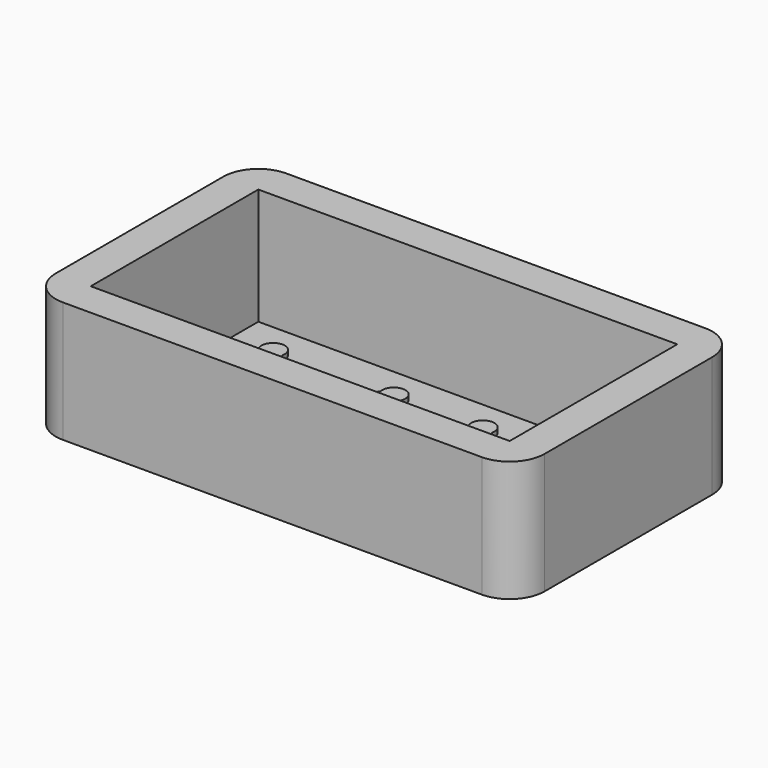
from build123d import *

# Parameters (mm, degrees)
F0_W     = 17.75
F0_H     = 18
F0_W_2   = 0.25
F1_DEPTH = 0.4
F2_DEPTH = 10
F3_DEPTH = 0.2
F4_DEPTH = 0.4


# Not quite as in the source:
# - a feature names something its author has since deleted; it is built from what else it names


with BuildPart() as f1:
    # F0 (on Top) → F1 (new body)
    with BuildSketch(Plane.XY):
        with BuildLine():
            Line((36, 21), (0, 21))
            ThreePointArc((0, 21), (-2.1213203436, 20.1213203436), (-3, 18))
            Line((-3, 18), (-3, 0))
            ThreePointArc((-3, 0), (-2.1213203436, -2.1213203436), (0, -3))
            Line((0, -3), (36, -3))
            ThreePointArc((36, -3), (38.1213203436, -2.1213203436), (39, 0))
            Line((39, 0), (39, 18))
            ThreePointArc((39, 18), (38.1213203436, 20.1213203436), (36, 21))
        make_face()
        Polygon((0, 0), (0, 18), (17.75, 18), (18, 18), (18.25, 18), (36, 18), (36, 0), (18.25, 0), (18, 0), (17.75, 0), align=None, mode=Mode.SUBTRACT)
        with Locations((8.875, 9)):
            Rectangle(F0_W, F0_H)
        with BuildLine():
            Line((9.6533412223, 11.6952957055), (9.9919033945, 10.9452957055))
            Line((9.9919033945, 10.9452957055), (10.3304655668, 11.6952957055))
            Line((10.3304655668, 11.6952957055), (10.9904227081, 12.3580254744))
            Line((10.9904227081, 12.3580254744), (13.2079580316, 14.5755632326))
            ThreePointArc((13.2079580316, 14.5755632326), (14.8809903029, 15.5414897832), (13.9150646707, 13.8684569817))
            Line((13.9150646707, 13.8684569817), (10.9919033945, 10.9452957055))
            Line((10.9919033945, 10.9452957055), (10.9919033945, 9.4452957055))
            Line((10.9919033945, 9.4452957055), (13.6148667214, 9.4452957055))
            ThreePointArc((13.6148667214, 9.4452957055), (13.70376764, 9.5296679116), (13.8052234095, 9.5984339593))
            ThreePointArc((13.8052234095, 9.5984339593), (14.9138690208, 8.823141097), (13.6148667214, 8.4452957055))
            Line((13.6148667214, 8.4452957055), (10.9919033945, 8.4452957055))
            Line((10.9919033945, 8.4452957055), (10.9919033945, 6.9452957055))
            Line((10.9919033945, 6.9452957055), (13.9150646707, 4.0221344294))
            ThreePointArc((13.9150646707, 4.0221344294), (14.8809903029, 2.3491016278), (13.2079580316, 3.3150281785))
            Line((13.2079580316, 3.3150281785), (10.9904227081, 5.5325659367))
            Line((10.9904227081, 5.5325659367), (10.3304655668, 6.1952957055))
            Line((10.3304655668, 6.1952957055), (9.9919033945, 6.9452957055))
            Line((9.9919033945, 6.9452957055), (9.6533412223, 6.1952957055))
            ThreePointArc((9.6533412223, 6.1952957055), (8.9919033945, 4.4452957055), (8.3304655668, 6.1952957055))
            Line((8.3304655668, 6.1952957055), (7.9919033945, 6.9452957055))
            Line((7.9919033945, 6.9452957055), (7.6533412223, 6.1952957055))
            Line((7.6533412223, 6.1952957055), (6.993384081, 5.5325659367))
            Line((6.993384081, 5.5325659367), (4.7758487575, 3.3150281785))
            ThreePointArc((4.7758487575, 3.3150281785), (3.1028164862, 2.3491016278), (4.0687421184, 4.0221344294))
            Line((4.0687421184, 4.0221344294), (6.9919033945, 6.9452957055))
            Line((6.9919033945, 6.9452957055), (6.9919033945, 8.4452957055))
            Line((6.9919033945, 8.4452957055), (4.3689400677, 8.4452957055))
            ThreePointArc((4.3689400677, 8.4452957055), (3.0699377683, 8.823141097), (4.1785833795, 9.5984339593))
            ThreePointArc((4.1785833795, 9.5984339593), (4.2800391491, 9.5296679116), (4.3689400677, 9.4452957055))
            Line((4.3689400677, 9.4452957055), (6.9919033945, 9.4452957055))
            Line((6.9919033945, 9.4452957055), (6.9919033945, 10.9452957055))
            Line((6.9919033945, 10.9452957055), (4.0687421184, 13.8684569817))
            ThreePointArc((4.0687421184, 13.8684569817), (3.1028164862, 15.5414897832), (4.7758487575, 14.5755632326))
            Line((4.7758487575, 14.5755632326), (6.993384081, 12.3580254744))
            Line((6.993384081, 12.3580254744), (7.6533412223, 11.6952957055))
            Line((7.6533412223, 11.6952957055), (7.9919033945, 10.9452957055))
            Line((7.9919033945, 10.9452957055), (8.3304655668, 11.6952957055))
            ThreePointArc((8.3304655668, 11.6952957055), (8.9919033945, 13.4452957055), (9.6533412223, 11.6952957055))
        make_face(mode=Mode.SUBTRACT)
        with Locations((27.125, 9)):
            Rectangle(F0_W, F0_H)
        with BuildLine():
            Line((27.6695344332, 11.6952957055), (28.0080966055, 10.9452957055))
            Line((28.0080966055, 10.9452957055), (28.3466587777, 11.6952957055))
            Line((28.3466587777, 11.6952957055), (29.006615919, 12.3580254744))
            Line((29.006615919, 12.3580254744), (31.2241512425, 14.5755632326))
            ThreePointArc((31.2241512425, 14.5755632326), (32.8971835138, 15.5414897832), (31.9312578816, 13.8684569817))
            Line((31.9312578816, 13.8684569817), (29.0080966055, 10.9452957055))
            Line((29.0080966055, 10.9452957055), (29.0080966055, 9.4452957055))
            Line((29.0080966055, 9.4452957055), (31.6310599323, 9.4452957055))
            ThreePointArc((31.6310599323, 9.4452957055), (31.7199608509, 9.5296679116), (31.8214166205, 9.5984339593))
            ThreePointArc((31.8214166205, 9.5984339593), (32.9300622317, 8.823141097), (31.6310599323, 8.4452957055))
            Line((31.6310599323, 8.4452957055), (29.0080966055, 8.4452957055))
            Line((29.0080966055, 8.4452957055), (29.0080966055, 6.9452957055))
            Line((29.0080966055, 6.9452957055), (31.9312578816, 4.0221344294))
            ThreePointArc((31.9312578816, 4.0221344294), (32.8971835138, 2.3491016278), (31.2241512425, 3.3150281785))
            Line((31.2241512425, 3.3150281785), (29.006615919, 5.5325659367))
            Line((29.006615919, 5.5325659367), (28.3466587777, 6.1952957055))
            Line((28.3466587777, 6.1952957055), (28.0080966055, 6.9452957055))
            Line((28.0080966055, 6.9452957055), (27.6695344332, 6.1952957055))
            ThreePointArc((27.6695344332, 6.1952957055), (27.0080966055, 4.4452957055), (26.3466587777, 6.1952957055))
            Line((26.3466587777, 6.1952957055), (26.0080966055, 6.9452957055))
            Line((26.0080966055, 6.9452957055), (25.6695344332, 6.1952957055))
            Line((25.6695344332, 6.1952957055), (25.0095772919, 5.5325659367))
            Line((25.0095772919, 5.5325659367), (22.7920419684, 3.3150281785))
            ThreePointArc((22.7920419684, 3.3150281785), (21.1190096971, 2.3491016278), (22.0849353293, 4.0221344294))
            Line((22.0849353293, 4.0221344294), (25.0080966055, 6.9452957055))
            Line((25.0080966055, 6.9452957055), (25.0080966055, 8.4452957055))
            Line((25.0080966055, 8.4452957055), (22.3851332786, 8.4452957055))
            ThreePointArc((22.3851332786, 8.4452957055), (21.0861309792, 8.823141097), (22.1947765905, 9.5984339593))
            ThreePointArc((22.1947765905, 9.5984339593), (22.29623236, 9.5296679116), (22.3851332786, 9.4452957055))
            Line((22.3851332786, 9.4452957055), (25.0080966055, 9.4452957055))
            Line((25.0080966055, 9.4452957055), (25.0080966055, 10.9452957055))
            Line((25.0080966055, 10.9452957055), (22.0849353293, 13.8684569817))
            ThreePointArc((22.0849353293, 13.8684569817), (21.1190096971, 15.5414897832), (22.7920419684, 14.5755632326))
            Line((22.7920419684, 14.5755632326), (25.0095772919, 12.3580254744))
            Line((25.0095772919, 12.3580254744), (25.6695344332, 11.6952957055))
            Line((25.6695344332, 11.6952957055), (26.0080966055, 10.9452957055))
            Line((26.0080966055, 10.9452957055), (26.3466587777, 11.6952957055))
            ThreePointArc((26.3466587777, 11.6952957055), (27.0080966055, 13.4452957055), (27.6695344332, 11.6952957055))
        make_face(mode=Mode.SUBTRACT)
        with BuildLine():
            Line((26.0080966055, 8.9452957055), (26.0080966055, 10.9452957055))
            Line((26.0080966055, 10.9452957055), (25.6695344332, 11.6952957055))
            Line((25.6695344332, 11.6952957055), (25.0095772919, 12.3580254744))
            Line((25.0095772919, 12.3580254744), (22.7920419684, 14.5755632326))
            ThreePointArc((22.7920419684, 14.5755632326), (21.1190096971, 15.5414897832), (22.0849353293, 13.8684569817))
            Line((22.0849353293, 13.8684569817), (25.0080966055, 10.9452957055))
            Line((25.0080966055, 10.9452957055), (25.0080966055, 9.4452957055))
            Line((25.0080966055, 9.4452957055), (25.0080966055, 8.9452957055))
            Line((25.0080966055, 8.9452957055), (25.0080966055, 8.4452957055))
            Line((25.0080966055, 8.4452957055), (25.0080966055, 6.9452957055))
            Line((25.0080966055, 6.9452957055), (22.0849353293, 4.0221344294))
            ThreePointArc((22.0849353293, 4.0221344294), (21.1190096971, 2.3491016278), (22.7920419684, 3.3150281785))
            Line((22.7920419684, 3.3150281785), (25.0095772919, 5.5325659367))
            Line((25.0095772919, 5.5325659367), (25.6695344332, 6.1952957055))
            Line((25.6695344332, 6.1952957055), (26.0080966055, 6.9452957055))
            Line((26.0080966055, 6.9452957055), (26.0080966055, 8.9452957055))
        make_face()
        with BuildLine():
            Line((28.3466587777, 11.6952957055), (28.0080966055, 10.9452957055))
            Line((28.0080966055, 10.9452957055), (28.0080966055, 8.9452957055))
            Line((28.0080966055, 8.9452957055), (28.0080966055, 6.9452957055))
            Line((28.0080966055, 6.9452957055), (28.3466587777, 6.1952957055))
            Line((28.3466587777, 6.1952957055), (29.006615919, 5.5325659367))
            Line((29.006615919, 5.5325659367), (31.2241512425, 3.3150281785))
            ThreePointArc((31.2241512425, 3.3150281785), (32.8971835138, 2.3491016278), (31.9312578816, 4.0221344294))
            Line((31.9312578816, 4.0221344294), (29.0080966055, 6.9452957055))
            Line((29.0080966055, 6.9452957055), (29.0080966055, 8.4452957055))
            Line((29.0080966055, 8.4452957055), (29.0080966055, 8.9452957055))
            Line((29.0080966055, 8.9452957055), (29.0080966055, 9.4452957055))
            Line((29.0080966055, 9.4452957055), (29.0080966055, 10.9452957055))
            Line((29.0080966055, 10.9452957055), (31.9312578816, 13.8684569817))
            ThreePointArc((31.9312578816, 13.8684569817), (32.8971835138, 15.5414897832), (31.2241512425, 14.5755632326))
            Line((31.2241512425, 14.5755632326), (29.006615919, 12.3580254744))
            Line((29.006615919, 12.3580254744), (28.3466587777, 11.6952957055))
        make_face()
        with BuildLine():
            Line((7.9919033945, 8.9452957055), (7.9919033945, 10.9452957055))
            Line((7.9919033945, 10.9452957055), (7.6533412223, 11.6952957055))
            Line((7.6533412223, 11.6952957055), (6.993384081, 12.3580254744))
            Line((6.993384081, 12.3580254744), (4.7758487575, 14.5755632326))
            ThreePointArc((4.7758487575, 14.5755632326), (3.1028164862, 15.5414897832), (4.0687421184, 13.8684569817))
            Line((4.0687421184, 13.8684569817), (6.9919033945, 10.9452957055))
            Line((6.9919033945, 10.9452957055), (6.9919033945, 9.4452957055))
            Line((6.9919033945, 9.4452957055), (6.9919033945, 8.9452957055))
            Line((6.9919033945, 8.9452957055), (6.9919033945, 8.4452957055))
            Line((6.9919033945, 8.4452957055), (6.9919033945, 6.9452957055))
            Line((6.9919033945, 6.9452957055), (4.0687421184, 4.0221344294))
            ThreePointArc((4.0687421184, 4.0221344294), (3.1028164862, 2.3491016278), (4.7758487575, 3.3150281785))
            Line((4.7758487575, 3.3150281785), (6.993384081, 5.5325659367))
            Line((6.993384081, 5.5325659367), (7.6533412223, 6.1952957055))
            Line((7.6533412223, 6.1952957055), (7.9919033945, 6.9452957055))
            Line((7.9919033945, 6.9452957055), (7.9919033945, 8.9452957055))
        make_face()
        with BuildLine():
            Line((9.9919033945, 10.9452957055), (9.9919033945, 8.9452957055))
            Line((9.9919033945, 8.9452957055), (9.9919033945, 6.9452957055))
            Line((9.9919033945, 6.9452957055), (10.3304655668, 6.1952957055))
            Line((10.3304655668, 6.1952957055), (10.9904227081, 5.5325659367))
            Line((10.9904227081, 5.5325659367), (13.2079580316, 3.3150281785))
            ThreePointArc((13.2079580316, 3.3150281785), (14.8809903029, 2.3491016278), (13.9150646707, 4.0221344294))
            Line((13.9150646707, 4.0221344294), (10.9919033945, 6.9452957055))
            Line((10.9919033945, 6.9452957055), (10.9919033945, 8.4452957055))
            Line((10.9919033945, 8.4452957055), (10.9919033945, 8.9452957055))
            Line((10.9919033945, 8.9452957055), (10.9919033945, 9.4452957055))
            Line((10.9919033945, 9.4452957055), (10.9919033945, 10.9452957055))
            Line((10.9919033945, 10.9452957055), (13.9150646707, 13.8684569817))
            ThreePointArc((13.9150646707, 13.8684569817), (14.8809903029, 15.5414897832), (13.2079580316, 14.5755632326))
            Line((13.2079580316, 14.5755632326), (10.9904227081, 12.3580254744))
            Line((10.9904227081, 12.3580254744), (10.3304655668, 11.6952957055))
            Line((10.3304655668, 11.6952957055), (9.9919033945, 10.9452957055))
        make_face()
        with BuildLine():
            Line((28.0080966055, 8.9452957055), (28.0080966055, 10.9452957055))
            Line((28.0080966055, 10.9452957055), (27.6695344332, 11.6952957055))
            ThreePointArc((27.6695344332, 11.6952957055), (27.0080966055, 13.4452957055), (26.3466587777, 11.6952957055))
            Line((26.3466587777, 11.6952957055), (26.0080966055, 10.9452957055))
            Line((26.0080966055, 10.9452957055), (26.0080966055, 8.9452957055))
            Line((26.0080966055, 8.9452957055), (26.0080966055, 6.9452957055))
            Line((26.0080966055, 6.9452957055), (26.3466587777, 6.1952957055))
            ThreePointArc((26.3466587777, 6.1952957055), (27.0080966055, 4.4452957055), (27.6695344332, 6.1952957055))
            Line((27.6695344332, 6.1952957055), (28.0080966055, 6.9452957055))
            Line((28.0080966055, 6.9452957055), (28.0080966055, 8.9452957055))
        make_face()
        with BuildLine():
            ThreePointArc((27.0080966055, 9.1952957055), (27.1848733008, 9.1220724008), (27.2580966055, 8.9452957055))
            ThreePointArc((27.2580966055, 8.9452957055), (27.1848733008, 8.7685190102), (27.0080966055, 8.6952957055))
            ThreePointArc((27.0080966055, 8.6952957055), (26.7580966055, 8.9452957055), (27.0080966055, 9.1952957055))
        make_face(mode=Mode.SUBTRACT)
        with BuildLine():
            Line((9.9919033945, 6.9452957055), (9.9919033945, 8.9452957055))
            Line((9.9919033945, 8.9452957055), (9.9919033945, 10.9452957055))
            Line((9.9919033945, 10.9452957055), (9.6533412223, 11.6952957055))
            ThreePointArc((9.6533412223, 11.6952957055), (8.9919033945, 13.4452957055), (8.3304655668, 11.6952957055))
            Line((8.3304655668, 11.6952957055), (7.9919033945, 10.9452957055))
            Line((7.9919033945, 10.9452957055), (7.9919033945, 8.9452957055))
            Line((7.9919033945, 8.9452957055), (7.9919033945, 6.9452957055))
            Line((7.9919033945, 6.9452957055), (8.3304655668, 6.1952957055))
            ThreePointArc((8.3304655668, 6.1952957055), (8.9919033945, 4.4452957055), (9.6533412223, 6.1952957055))
            Line((9.6533412223, 6.1952957055), (9.9919033945, 6.9452957055))
        make_face()
        with BuildLine():
            ThreePointArc((8.9919033945, 9.1952957055), (9.1686800898, 9.1220724008), (9.2419033945, 8.9452957055))
            ThreePointArc((9.2419033945, 8.9452957055), (9.1686800898, 8.7685190102), (8.9919033945, 8.6952957055))
            ThreePointArc((8.9919033945, 8.6952957055), (8.7419033945, 8.9452957055), (8.9919033945, 9.1952957055))
        make_face(mode=Mode.SUBTRACT)
        with Locations((17.875, 9)):
            Rectangle(F0_W_2, F0_H)
        with Locations((18.125, 9)):
            Rectangle(F0_W_2, F0_H)
        with BuildLine():
            Line((6.9919033945, 8.9452957055), (6.9919033945, 9.4452957055))
            Line((6.9919033945, 9.4452957055), (4.3689400677, 9.4452957055))
            ThreePointArc((4.3689400677, 9.4452957055), (4.2800391491, 9.5296679116), (4.1785833795, 9.5984339593))
            ThreePointArc((4.1785833795, 9.5984339593), (3.0699377683, 8.823141097), (4.3689400677, 8.4452957055))
            Line((4.3689400677, 8.4452957055), (6.9919033945, 8.4452957055))
            Line((6.9919033945, 8.4452957055), (6.9919033945, 8.9452957055))
        make_face()
        with BuildLine():
            Line((31.6310599323, 9.4452957055), (29.0080966055, 9.4452957055))
            Line((29.0080966055, 9.4452957055), (29.0080966055, 8.9452957055))
            Line((29.0080966055, 8.9452957055), (29.0080966055, 8.4452957055))
            Line((29.0080966055, 8.4452957055), (31.6310599323, 8.4452957055))
            ThreePointArc((31.6310599323, 8.4452957055), (32.9300622317, 8.823141097), (31.8214166205, 9.5984339593))
            ThreePointArc((31.8214166205, 9.5984339593), (31.7199608509, 9.5296679116), (31.6310599323, 9.4452957055))
        make_face()
        with BuildLine():
            Line((25.0080966055, 8.9452957055), (25.0080966055, 9.4452957055))
            Line((25.0080966055, 9.4452957055), (22.3851332786, 9.4452957055))
            ThreePointArc((22.3851332786, 9.4452957055), (22.29623236, 9.5296679116), (22.1947765905, 9.5984339593))
            ThreePointArc((22.1947765905, 9.5984339593), (21.0861309792, 8.823141097), (22.3851332786, 8.4452957055))
            Line((22.3851332786, 8.4452957055), (25.0080966055, 8.4452957055))
            Line((25.0080966055, 8.4452957055), (25.0080966055, 8.9452957055))
        make_face()
        with BuildLine():
            Line((13.6148667214, 9.4452957055), (10.9919033945, 9.4452957055))
            Line((10.9919033945, 9.4452957055), (10.9919033945, 8.9452957055))
            Line((10.9919033945, 8.9452957055), (10.9919033945, 8.4452957055))
            Line((10.9919033945, 8.4452957055), (13.6148667214, 8.4452957055))
            ThreePointArc((13.6148667214, 8.4452957055), (14.9138690208, 8.823141097), (13.8052234095, 9.5984339593))
            ThreePointArc((13.8052234095, 9.5984339593), (13.70376764, 9.5296679116), (13.6148667214, 9.4452957055))
        make_face()
        with BuildLine():
            ThreePointArc((8.9919033945, 8.6952957055), (9.1686800898, 8.7685190102), (9.2419033945, 8.9452957055))
            ThreePointArc((9.2419033945, 8.9452957055), (9.1686800898, 9.1220724008), (8.9919033945, 9.1952957055))
            Line((8.9919033945, 9.1952957055), (8.9919033945, 8.6952957055))
        make_face()
        with BuildLine():
            ThreePointArc((27.0080966055, 8.6952957055), (27.1848733008, 8.7685190102), (27.2580966055, 8.9452957055))
            ThreePointArc((27.2580966055, 8.9452957055), (27.1848733008, 9.1220724008), (27.0080966055, 9.1952957055))
            Line((27.0080966055, 9.1952957055), (27.0080966055, 8.6952957055))
        make_face()
        with BuildLine():
            Line((8.9919033945, 8.6952957055), (8.9919033945, 9.1952957055))
            ThreePointArc((8.9919033945, 9.1952957055), (8.7419033945, 8.9452957055), (8.9919033945, 8.6952957055))
        make_face()
        with BuildLine():
            Line((27.0080966055, 8.6952957055), (27.0080966055, 9.1952957055))
            ThreePointArc((27.0080966055, 9.1952957055), (26.7580966055, 8.9452957055), (27.0080966055, 8.6952957055))
        make_face()
    extrude(amount=-F1_DEPTH)

    # F0 (on Top) → F2 (join)
    with BuildSketch(Plane.XY):
        with BuildLine():
            Line((36, 21), (0, 21))
            ThreePointArc((0, 21), (-2.1213203436, 20.1213203436), (-3, 18))
            Line((-3, 18), (-3, 0))
            ThreePointArc((-3, 0), (-2.1213203436, -2.1213203436), (0, -3))
            Line((0, -3), (36, -3))
            ThreePointArc((36, -3), (38.1213203436, -2.1213203436), (39, 0))
            Line((39, 0), (39, 18))
            ThreePointArc((39, 18), (38.1213203436, 20.1213203436), (36, 21))
        make_face()
        Polygon((0, 0), (0, 18), (17.75, 18), (18, 18), (18.25, 18), (36, 18), (36, 0), (18.25, 0), (18, 0), (17.75, 0), align=None, mode=Mode.SUBTRACT)
    extrude(amount=F2_DEPTH)

    # F0 (on Top) → F3 (join)
    with BuildSketch(Plane.XY):
        with BuildLine():
            Line((9.9919033945, 6.9452957055), (9.9919033945, 8.9452957055))
            Line((9.9919033945, 8.9452957055), (9.9919033945, 10.9452957055))
            Line((9.9919033945, 10.9452957055), (9.6533412223, 11.6952957055))
            ThreePointArc((9.6533412223, 11.6952957055), (8.9919033945, 13.4452957055), (8.3304655668, 11.6952957055))
            Line((8.3304655668, 11.6952957055), (7.9919033945, 10.9452957055))
            Line((7.9919033945, 10.9452957055), (7.9919033945, 8.9452957055))
            Line((7.9919033945, 8.9452957055), (7.9919033945, 6.9452957055))
            Line((7.9919033945, 6.9452957055), (8.3304655668, 6.1952957055))
            ThreePointArc((8.3304655668, 6.1952957055), (8.9919033945, 4.4452957055), (9.6533412223, 6.1952957055))
            Line((9.6533412223, 6.1952957055), (9.9919033945, 6.9452957055))
        make_face()
        with BuildLine():
            ThreePointArc((8.9919033945, 9.1952957055), (9.1686800898, 9.1220724008), (9.2419033945, 8.9452957055))
            ThreePointArc((9.2419033945, 8.9452957055), (9.1686800898, 8.7685190102), (8.9919033945, 8.6952957055))
            ThreePointArc((8.9919033945, 8.6952957055), (8.7419033945, 8.9452957055), (8.9919033945, 9.1952957055))
        make_face(mode=Mode.SUBTRACT)
        with BuildLine():
            Line((13.6148667214, 9.4452957055), (10.9919033945, 9.4452957055))
            Line((10.9919033945, 9.4452957055), (10.9919033945, 8.9452957055))
            Line((10.9919033945, 8.9452957055), (10.9919033945, 8.4452957055))
            Line((10.9919033945, 8.4452957055), (13.6148667214, 8.4452957055))
            ThreePointArc((13.6148667214, 8.4452957055), (14.9138690208, 8.823141097), (13.8052234095, 9.5984339593))
            ThreePointArc((13.8052234095, 9.5984339593), (13.70376764, 9.5296679116), (13.6148667214, 9.4452957055))
        make_face()
        with BuildLine():
            Line((6.9919033945, 8.9452957055), (6.9919033945, 9.4452957055))
            Line((6.9919033945, 9.4452957055), (4.3689400677, 9.4452957055))
            ThreePointArc((4.3689400677, 9.4452957055), (4.2800391491, 9.5296679116), (4.1785833795, 9.5984339593))
            ThreePointArc((4.1785833795, 9.5984339593), (3.0699377683, 8.823141097), (4.3689400677, 8.4452957055))
            Line((4.3689400677, 8.4452957055), (6.9919033945, 8.4452957055))
            Line((6.9919033945, 8.4452957055), (6.9919033945, 8.9452957055))
        make_face()
        with BuildLine():
            Line((25.0080966055, 8.9452957055), (25.0080966055, 9.4452957055))
            Line((25.0080966055, 9.4452957055), (22.3851332786, 9.4452957055))
            ThreePointArc((22.3851332786, 9.4452957055), (22.29623236, 9.5296679116), (22.1947765905, 9.5984339593))
            ThreePointArc((22.1947765905, 9.5984339593), (21.0861309792, 8.823141097), (22.3851332786, 8.4452957055))
            Line((22.3851332786, 8.4452957055), (25.0080966055, 8.4452957055))
            Line((25.0080966055, 8.4452957055), (25.0080966055, 8.9452957055))
        make_face()
        with BuildLine():
            Line((28.0080966055, 8.9452957055), (28.0080966055, 10.9452957055))
            Line((28.0080966055, 10.9452957055), (27.6695344332, 11.6952957055))
            ThreePointArc((27.6695344332, 11.6952957055), (27.0080966055, 13.4452957055), (26.3466587777, 11.6952957055))
            Line((26.3466587777, 11.6952957055), (26.0080966055, 10.9452957055))
            Line((26.0080966055, 10.9452957055), (26.0080966055, 8.9452957055))
            Line((26.0080966055, 8.9452957055), (26.0080966055, 6.9452957055))
            Line((26.0080966055, 6.9452957055), (26.3466587777, 6.1952957055))
            ThreePointArc((26.3466587777, 6.1952957055), (27.0080966055, 4.4452957055), (27.6695344332, 6.1952957055))
            Line((27.6695344332, 6.1952957055), (28.0080966055, 6.9452957055))
            Line((28.0080966055, 6.9452957055), (28.0080966055, 8.9452957055))
        make_face()
        with BuildLine():
            ThreePointArc((27.0080966055, 9.1952957055), (27.1848733008, 9.1220724008), (27.2580966055, 8.9452957055))
            ThreePointArc((27.2580966055, 8.9452957055), (27.1848733008, 8.7685190102), (27.0080966055, 8.6952957055))
            ThreePointArc((27.0080966055, 8.6952957055), (26.7580966055, 8.9452957055), (27.0080966055, 9.1952957055))
        make_face(mode=Mode.SUBTRACT)
        with BuildLine():
            Line((31.6310599323, 9.4452957055), (29.0080966055, 9.4452957055))
            Line((29.0080966055, 9.4452957055), (29.0080966055, 8.9452957055))
            Line((29.0080966055, 8.9452957055), (29.0080966055, 8.4452957055))
            Line((29.0080966055, 8.4452957055), (31.6310599323, 8.4452957055))
            ThreePointArc((31.6310599323, 8.4452957055), (32.9300622317, 8.823141097), (31.8214166205, 9.5984339593))
            ThreePointArc((31.8214166205, 9.5984339593), (31.7199608509, 9.5296679116), (31.6310599323, 9.4452957055))
        make_face()
    extrude(amount=F3_DEPTH)

    # F0 (on Top) → F4 (join)
    with BuildSketch(Plane.XY):
        with BuildLine():
            Line((7.9919033945, 8.9452957055), (7.9919033945, 10.9452957055))
            Line((7.9919033945, 10.9452957055), (7.6533412223, 11.6952957055))
            Line((7.6533412223, 11.6952957055), (6.993384081, 12.3580254744))
            Line((6.993384081, 12.3580254744), (4.7758487575, 14.5755632326))
            ThreePointArc((4.7758487575, 14.5755632326), (3.1028164862, 15.5414897832), (4.0687421184, 13.8684569817))
            Line((4.0687421184, 13.8684569817), (6.9919033945, 10.9452957055))
            Line((6.9919033945, 10.9452957055), (6.9919033945, 9.4452957055))
            Line((6.9919033945, 9.4452957055), (6.9919033945, 8.9452957055))
            Line((6.9919033945, 8.9452957055), (6.9919033945, 8.4452957055))
            Line((6.9919033945, 8.4452957055), (6.9919033945, 6.9452957055))
            Line((6.9919033945, 6.9452957055), (4.0687421184, 4.0221344294))
            ThreePointArc((4.0687421184, 4.0221344294), (3.1028164862, 2.3491016278), (4.7758487575, 3.3150281785))
            Line((4.7758487575, 3.3150281785), (6.993384081, 5.5325659367))
            Line((6.993384081, 5.5325659367), (7.6533412223, 6.1952957055))
            Line((7.6533412223, 6.1952957055), (7.9919033945, 6.9452957055))
            Line((7.9919033945, 6.9452957055), (7.9919033945, 8.9452957055))
        make_face()
        with BuildLine():
            Line((9.9919033945, 10.9452957055), (9.9919033945, 8.9452957055))
            Line((9.9919033945, 8.9452957055), (9.9919033945, 6.9452957055))
            Line((9.9919033945, 6.9452957055), (10.3304655668, 6.1952957055))
            Line((10.3304655668, 6.1952957055), (10.9904227081, 5.5325659367))
            Line((10.9904227081, 5.5325659367), (13.2079580316, 3.3150281785))
            ThreePointArc((13.2079580316, 3.3150281785), (14.8809903029, 2.3491016278), (13.9150646707, 4.0221344294))
            Line((13.9150646707, 4.0221344294), (10.9919033945, 6.9452957055))
            Line((10.9919033945, 6.9452957055), (10.9919033945, 8.4452957055))
            Line((10.9919033945, 8.4452957055), (10.9919033945, 8.9452957055))
            Line((10.9919033945, 8.9452957055), (10.9919033945, 9.4452957055))
            Line((10.9919033945, 9.4452957055), (10.9919033945, 10.9452957055))
            Line((10.9919033945, 10.9452957055), (13.9150646707, 13.8684569817))
            ThreePointArc((13.9150646707, 13.8684569817), (14.8809903029, 15.5414897832), (13.2079580316, 14.5755632326))
            Line((13.2079580316, 14.5755632326), (10.9904227081, 12.3580254744))
            Line((10.9904227081, 12.3580254744), (10.3304655668, 11.6952957055))
            Line((10.3304655668, 11.6952957055), (9.9919033945, 10.9452957055))
        make_face()
        with BuildLine():
            Line((26.0080966055, 8.9452957055), (26.0080966055, 10.9452957055))
            Line((26.0080966055, 10.9452957055), (25.6695344332, 11.6952957055))
            Line((25.6695344332, 11.6952957055), (25.0095772919, 12.3580254744))
            Line((25.0095772919, 12.3580254744), (22.7920419684, 14.5755632326))
            ThreePointArc((22.7920419684, 14.5755632326), (21.1190096971, 15.5414897832), (22.0849353293, 13.8684569817))
            Line((22.0849353293, 13.8684569817), (25.0080966055, 10.9452957055))
            Line((25.0080966055, 10.9452957055), (25.0080966055, 9.4452957055))
            Line((25.0080966055, 9.4452957055), (25.0080966055, 8.9452957055))
            Line((25.0080966055, 8.9452957055), (25.0080966055, 8.4452957055))
            Line((25.0080966055, 8.4452957055), (25.0080966055, 6.9452957055))
            Line((25.0080966055, 6.9452957055), (22.0849353293, 4.0221344294))
            ThreePointArc((22.0849353293, 4.0221344294), (21.1190096971, 2.3491016278), (22.7920419684, 3.3150281785))
            Line((22.7920419684, 3.3150281785), (25.0095772919, 5.5325659367))
            Line((25.0095772919, 5.5325659367), (25.6695344332, 6.1952957055))
            Line((25.6695344332, 6.1952957055), (26.0080966055, 6.9452957055))
            Line((26.0080966055, 6.9452957055), (26.0080966055, 8.9452957055))
        make_face()
        with BuildLine():
            Line((28.3466587777, 11.6952957055), (28.0080966055, 10.9452957055))
            Line((28.0080966055, 10.9452957055), (28.0080966055, 8.9452957055))
            Line((28.0080966055, 8.9452957055), (28.0080966055, 6.9452957055))
            Line((28.0080966055, 6.9452957055), (28.3466587777, 6.1952957055))
            Line((28.3466587777, 6.1952957055), (29.006615919, 5.5325659367))
            Line((29.006615919, 5.5325659367), (31.2241512425, 3.3150281785))
            ThreePointArc((31.2241512425, 3.3150281785), (32.8971835138, 2.3491016278), (31.9312578816, 4.0221344294))
            Line((31.9312578816, 4.0221344294), (29.0080966055, 6.9452957055))
            Line((29.0080966055, 6.9452957055), (29.0080966055, 8.4452957055))
            Line((29.0080966055, 8.4452957055), (29.0080966055, 8.9452957055))
            Line((29.0080966055, 8.9452957055), (29.0080966055, 9.4452957055))
            Line((29.0080966055, 9.4452957055), (29.0080966055, 10.9452957055))
            Line((29.0080966055, 10.9452957055), (31.9312578816, 13.8684569817))
            ThreePointArc((31.9312578816, 13.8684569817), (32.8971835138, 15.5414897832), (31.2241512425, 14.5755632326))
            Line((31.2241512425, 14.5755632326), (29.006615919, 12.3580254744))
            Line((29.006615919, 12.3580254744), (28.3466587777, 11.6952957055))
        make_face()
    extrude(amount=F4_DEPTH)


solid = f1.part
